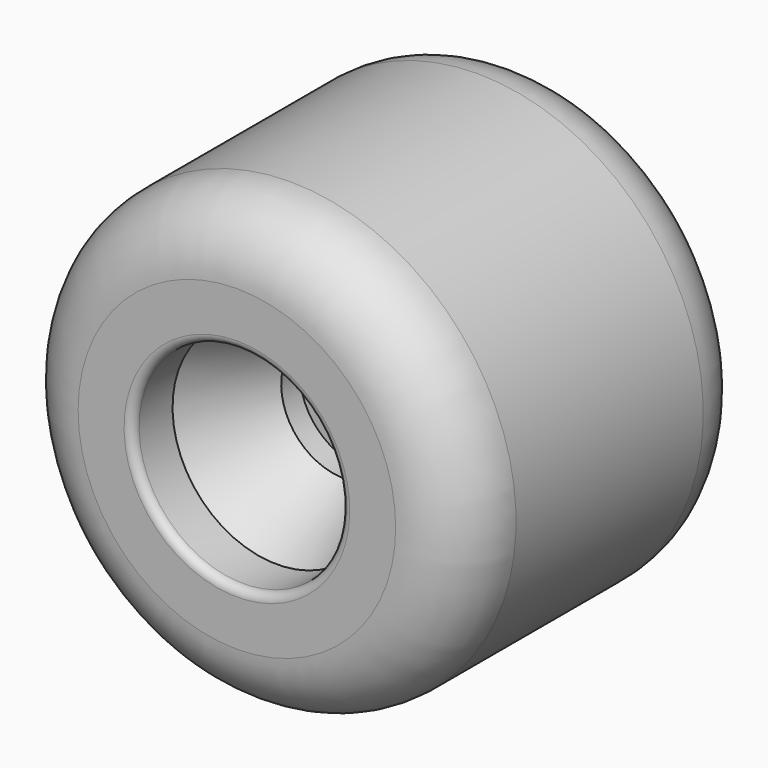
from build123d import *

# Parameters (mm, degrees)
F2_R     = 40
F3_R     = 5
F4_R     = 5
F5_R     = 4.25
F6_DEPTH = 10
F7_COUNT = 3


# Not quite as in the source:
# - a feature names something its author has since deleted; it is built from what else it names


with BuildPart() as f1:
    # F0 (on Right) → F1 (revolve)
    with BuildSketch(Plane.YZ):
        Polygon((115.0588170719, 135), (-104.9411829281, 135), (-104.9411829281, 62.5099688768), (-74.9411829281, 62.5099688768), (-24.9411829281, 37.5), (-10.9411829281, 37.5), (-10.9411829281, 20), (-0.9411829281, 20), (-0.9411829281, 37.5), (23.0588170719, 37.5), (65.0588170719, 58.5), (115.0588170719, 58.5), align=None)
    revolve(axis=Axis((0, 3.7167160804, 0), (0, -1, 0)))

    # F2
    f2_edges = [f1.edges().sort_by_distance(p)[0] for p in [
        (0, -104.941183, -135),
        (0, 115.058817, -135),
    ]]
    fillet(f2_edges, radius=F2_R)

    # F3
    f3_edges = [f1.edges().sort_by_distance(p)[0] for p in [
        (0, -104.941183, -62.509969),
    ]]
    fillet(f3_edges, radius=F3_R)

    # F4
    f4_edges = [f1.edges().sort_by_distance(p)[0] for p in [
        (0, 115.058817, -58.5),
    ]]
    fillet(f4_edges, radius=F4_R)

    # F5 (on face) → F6 (cut, through all)
    with BuildSketch(Plane.XZ.offset(10.9411829281)):
        with Locations((0, 29)):
            Circle(F5_R)
    f6 = extrude(amount=-F6_DEPTH, mode=Mode.SUBTRACT)

    # F7: F6 ×3 about axis
    f7_axis = Axis((0, 3.7167160804, 0), (0, -1, 0))
    for i in range(1, F7_COUNT):
        add(f6.rotate(f7_axis, i * 360 / F7_COUNT), mode=Mode.SUBTRACT)


solid = f1.part
